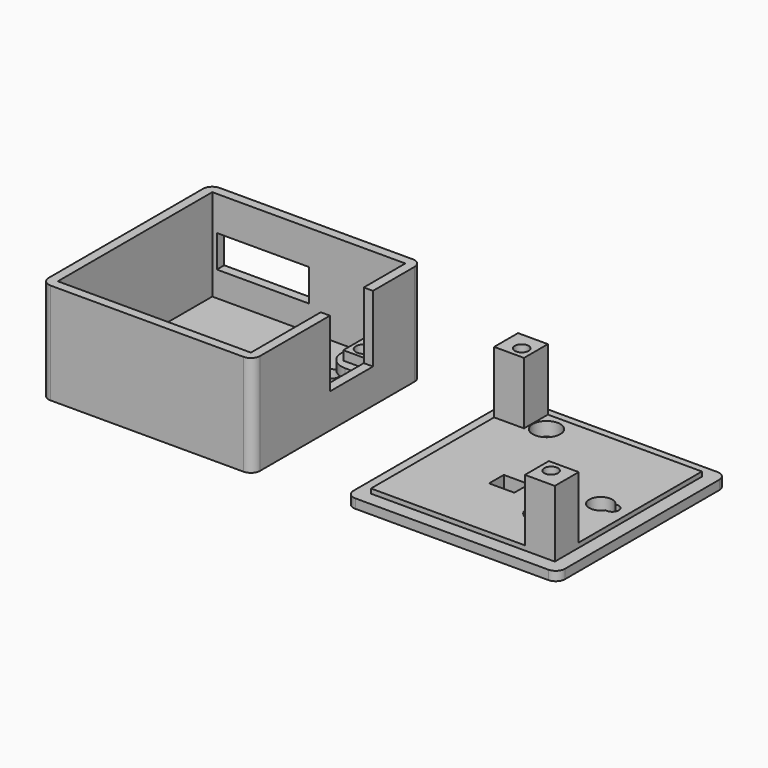
from build123d import *

# Parameters (mm, degrees)
F0_W         = 46
F0_H         = 46
F1_DEPTH     = 22
F2_W         = 42
F2_H         = 42
F3_DEPTH     = 20
F4_W         = 7.5
F4_H         = 7.5
F5_DEPTH     = 4
F7_W         = 2
F7_H         = 7.5
F8_DEPTH     = 2
F10_DEPTH    = 2
F11_W        = 46
F11_H        = 46
F12_DEPTH    = 2
F13_W        = 40
F13_H        = 40
F14_DEPTH    = 1
F15_W        = 6.5
F15_H        = 6.5
F16_DEPTH    = 13.5
F17_R        = 1.5
F18_DEPTH    = 25
F19_DEPTH    = 25
F20_W        = 11.7
F20_H        = 14.5
F21_DEPTH    = 2
F22_W        = 20
F22_H        = 7
F23_DEPTH    = 2
F24_R        = 3
F24_W        = 5.5
F24_H        = 4
F25_DEPTH    = 3
F26_W        = 14
F26_H        = 14
F26_R        = 1.75
F28_DEPTH    = 2
F27_R        = 2.5
F27_R_2      = 1.5
F29_DEPTH    = 1.5
F6_R         = 1.75
F30_DEPTH    = 25
F31_T1_DEPTH = 12
F32_R        = 2
F32_2_R      = 2


# Not quite as in the source:
# - a fillet or chamfer that OpenCascade refuses, or shapes differently, is made with other operations: its cross-section is extruded or revolved along the edge and cut away or added
# - a feature names something its author has since deleted; it is built from what else it names


with BuildPart() as f1:
    # F0 (on Top) → F1 (new body)
    with BuildSketch(Plane.XY):
        with Locations((-34.8121308275, 37.9456170828)):
            Rectangle(F0_W, F0_H)
    extrude(amount=F1_DEPTH)

    # F2 (on face) → F3 (cut)
    with BuildSketch(Plane.XY.offset(22)):
        with Locations((-34.8121308275, 37.9456170828)):
            Rectangle(F2_W, F2_H)
    extrude(amount=-F3_DEPTH, mode=Mode.SUBTRACT)

    # F4 (on face) → F5 (join)
    with BuildSketch(Plane.XY.offset(2)):
        with Locations((-52.0621308275, 20.6956170828)):
            Rectangle(F4_W, F4_H)
        with Locations((-17.5621308275, 55.1956170828)):
            Rectangle(F4_W, F4_H)
    extrude(amount=F5_DEPTH)

    # F7 (on face) → F8 (join)
    with BuildSketch(Plane.XY.offset(2)):
        Polygon((-46.3121308275, 26.4456170828), (-55.8121308275, 26.4456170828), (-55.8121308275, 24.4456170828), (-48.3121308275, 24.4456170828), (-46.3121308275, 24.4456170828), align=None)
        with Locations((-47.3121308275, 20.6956170828)):
            Rectangle(F7_W, F7_H)
        with Locations((-22.3121308275, 55.1956170828)):
            Rectangle(F7_W, F7_H)
        Polygon((-13.8121308275, 51.4456170828), (-21.3121308275, 51.4456170828), (-23.3121308275, 51.4456170828), (-23.3121308275, 49.4456170828), (-13.8121308275, 49.4456170828), align=None)
    extrude(amount=F8_DEPTH)

    # F9 (on face) → F10 (cut)
    with BuildSketch(Plane(origin=(0, 0, 0), x_dir=(1, 0, 0), z_dir=(0, 0, -1))):
        Polygon((-16.0621308275, -55.5333303231), (-16.0621308275, -52.3579038425), (-18.8121308275, -50.7701906023), (-21.5621308275, -52.3579038425), (-21.5621308275, -55.5333303231), (-18.8121308275, -57.1210435634), align=None)
        Polygon((-47.6367043469, -21.9456170828), (-49.2244175872, -19.1956170828), (-52.3998440677, -19.1956170828), (-53.987557308, -21.9456170828), (-52.3998440677, -24.6956170828), (-49.2244175872, -24.6956170828), align=None)
    extrude(amount=-F10_DEPTH, mode=Mode.SUBTRACT)

    # F20 (on face) → F21 (cut)
    with BuildSketch(Plane.YZ.offset(-11.8121308275)):
        with Locations((41.7956170828, 14.75)):
            Rectangle(F20_W, F20_H)
    extrude(amount=-F21_DEPTH, mode=Mode.SUBTRACT)

    # F22 (on face) → F23 (cut)
    with BuildSketch(Plane(origin=(0, 60.9456170828, 0), x_dir=(-1, 0, 0), z_dir=(0, 1, 0))):
        with Locations((44.8121308275, 11)):
            Rectangle(F22_W, F22_H)
    extrude(amount=-F23_DEPTH, mode=Mode.SUBTRACT)

    # F26 (on face) → F28 (cut)
    with BuildSketch(Plane(origin=(0, 0, 0), x_dir=(1, 0, 0), z_dir=(0, 0, -1))):
        with Locations((-36.8121308275, -26.9456170828)):
            Rectangle(F26_W, F26_H)
        with Locations((-22.3021308275, -49.3056170828)):
            Circle(F26_R)
    extrude(amount=-F28_DEPTH, mode=Mode.SUBTRACT)

    # F6 (on face) → F30 (cut)
    with BuildSketch(Plane.XY.offset(22)):
        with Locations((-18.8121308275, 53.9456170828)):
            Circle(F6_R)
        with Locations((-50.8121308275, 21.9456170828)):
            Circle(F6_R)
    extrude(amount=-F30_DEPTH, mode=Mode.SUBTRACT)

    # F31: fillet of radius 4 on 2 edges, made by hand

    # F31_s2 → F31_t1 (cut)
    with BuildSketch(Plane.XY.offset(2)):
        with BuildLine():
            ThreePointArc((-50.3121308275, 26.4456170828), (-47.4837037027, 25.2740442076), (-46.3121308275, 22.4456170828))
            Line((-46.3121308275, 22.4456170828), (-46.3121308275, 26.4456170828))
            Line((-46.3121308275, 26.4456170828), (-50.3121308275, 26.4456170828))
        make_face()
        with BuildLine():
            ThreePointArc((-19.3121308275, 49.4456170828), (-22.1405579522, 50.6171899581), (-23.3121308275, 53.4456170828))
            Line((-23.3121308275, 53.4456170828), (-23.3121308275, 49.4456170828))
            Line((-23.3121308275, 49.4456170828), (-19.3121308275, 49.4456170828))
        make_face()
    extrude(amount=F31_T1_DEPTH, mode=Mode.SUBTRACT)

    # F32
    f32_edges = [f1.edges().sort_by_distance(p)[0] for p in [
        (-57.812131, 14.945617, 11),
        (-57.812131, 60.945617, 11),
        (-11.812131, 60.945617, 11),
        (-11.812131, 14.945617, 11),
    ]]
    fillet(f32_edges, radius=F32_R)


with BuildPart() as f12:
    # F11 (on Top) → F12 (new body)
    with BuildSketch(Plane.XY):
        with Locations((30.5410524812, 39.1538485997)):
            Rectangle(F11_W, F11_H)
    extrude(amount=F12_DEPTH)

    # F13 (on face) → F14 (join)
    with BuildSketch(Plane.XY.offset(2)):
        with Locations((30.5410524812, 39.1538485997)):
            Rectangle(F13_W, F13_H)
    extrude(amount=F14_DEPTH)

    # F15 (on face) → F16 (join)
    with BuildSketch(Plane.XY.offset(3)):
        with Locations((13.7910524812, 55.9038485997)):
            Rectangle(F15_W, F15_H)
        with Locations((47.2910524812, 22.4038485997)):
            Rectangle(F15_W, F15_H)
    extrude(amount=F16_DEPTH)

    # F17 (on face) → F18 (cut)
    with BuildSketch(Plane.XY.offset(3)):
        with Locations((14.5410524812, 55.1538485997)):
            Circle(F17_R)
        with Locations((46.5410524812, 23.1538485997)):
            Circle(F17_R)
    extrude(amount=F18_DEPTH, mode=Mode.SUBTRACT)

    # F17 (on face) → F19 (cut)
    with BuildSketch(Plane.XY.offset(3)):
        with Locations((14.5410524812, 55.1538485997)):
            Circle(F17_R)
        with Locations((46.5410524812, 23.1538485997)):
            Circle(F17_R)
    extrude(amount=-F19_DEPTH, mode=Mode.SUBTRACT)

    # F24 (on face) → F25 (cut)
    with BuildSketch(Plane(origin=(0, 0, 0), x_dir=(1, 0, 0), z_dir=(0, 0, -1))):
        with Locations((38.8610524812, -29.9538485997)):
            Circle(F24_R)
        with Locations((27.7910524812, -35.1538485997)):
            Rectangle(F24_W, F24_H)
        with Locations((20.1910524812, -54.8338485997)):
            Circle(F24_R)
        with BuildLine():
            ThreePointArc((46.6490524812, -40.4978485997), (45.6410524812, -39.1538485997), (46.6490524812, -37.8098485997))
            ThreePointArc((46.6490524812, -37.8098485997), (42.0410524812, -39.1538485997), (46.6490524812, -40.4978485997))
        make_face()
        with BuildLine():
            ThreePointArc((46.6490524812, -37.8098485997), (46.9410524812, -38.4538485997), (47.0410524812, -39.1538485997))
            ThreePointArc((47.0410524812, -39.1538485997), (46.9410524812, -39.8538485997), (46.6490524812, -40.4978485997))
            ThreePointArc((46.6490524812, -40.4978485997), (47.8810524812, -40.2738485997), (48.4410524812, -39.1538485997))
            ThreePointArc((48.4410524812, -39.1538485997), (47.8810524812, -38.0338485997), (46.6490524812, -37.8098485997))
        make_face()
        with BuildLine():
            ThreePointArc((46.6490524812, -40.4978485997), (46.9410524812, -39.8538485997), (47.0410524812, -39.1538485997))
            ThreePointArc((47.0410524812, -39.1538485997), (46.9410524812, -38.4538485997), (46.6490524812, -37.8098485997))
            ThreePointArc((46.6490524812, -37.8098485997), (45.6410524812, -39.1538485997), (46.6490524812, -40.4978485997))
        make_face()
    extrude(amount=-F25_DEPTH, mode=Mode.SUBTRACT)

    # F27 (on face) → F29 (cut)
    with BuildSketch(Plane(origin=(0, 0, 0), x_dir=(1, 0, 0), z_dir=(0, 0, -1))):
        with Locations((14.5410524812, -55.1538485997)):
            Circle(F27_R)
        with Locations((14.5410524812, -55.1538485997)):
            Circle(F27_R_2, mode=Mode.SUBTRACT)
        with Locations((46.5410524812, -23.1538485997)):
            Circle(F27_R)
        with Locations((46.5410524812, -23.1538485997)):
            Circle(F27_R_2, mode=Mode.SUBTRACT)
    extrude(amount=-F29_DEPTH, mode=Mode.SUBTRACT)

    # F32#2
    f32_2_edges = [f12.edges().sort_by_distance(p)[0] for p in [
        (7.541052, 16.153849, 1),
        (7.541052, 62.153849, 1),
        (53.541052, 62.153849, 1),
        (53.541052, 16.153849, 1),
    ]]
    fillet(f32_2_edges, radius=F32_2_R)


solid = Compound([f1.part, f12.part])
